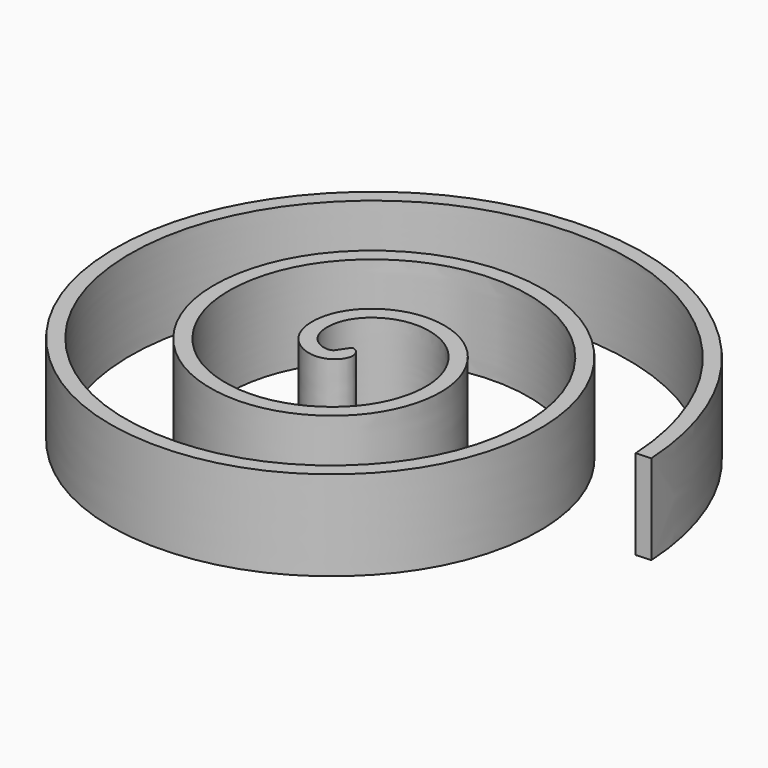
from build123d import *

# Parameters (mm, degrees)
F1_DEPTH = 3


# Not quite as in the source:
# - the dataset's text gives a spline's control points without its knots; the knots are read off the source's solid


with BuildPart() as f1:
    # F0 (on Top) → F1 (new body)
    with BuildSketch(Plane.XY):
        with BuildLine():
            Line((9.780739, 0.387732), (10.280037, 0.414221))
            add(Edge.make_bspline(
                [(10.280037, 0.414221), (10.201374, 1.896982), (9.787847, 3.342673), (7.912828, 6.782154), (5.908292, 8.419424), (1.404738, 9.873726), (-1.068266, 9.68826), (-5.152995, 7.729246), (-6.745094, 5.971338), (-8.285187, 1.926739), (-8.230102, -0.336088), (-6.637868, -4.142075), (-5.114518, -5.666794), (-1.522909, -7.245819), (0.523612, -7.296699), (4.02363, -6.032875), (5.460011, -4.730316), (7.03213, -1.581924), (7.164322, 0.244253), (6.1887, 3.414553), (5.091573, 4.743007), (2.372921, 6.26368), (0.769032, 6.452455), (-2.051397, 5.723262), (-3.253819, 4.81473), (-4.680076, 2.508754), (-4.900784, 1.127007), (-4.374962, -1.327091), (-3.636828, -2.386958), (-1.723014, -3.67766), (-0.561192, -3.905889), (1.513882, -3.53938), (2.41635, -2.952214), (3.53244, -1.406757), (3.74417, -0.4606), (3.492204, 1.226583), (3.035476, 1.958572), (1.831454, 2.863311), (1.094698, 3.035068), (-0.199589, 2.852457), (-0.749855, 2.504675), (-1.533897, 1.443211), (-1.550306, 0.6687), (-1.006795, -0.355611), (-0.483723, -0.590581), (0.31479, -0.499144), (0.565644, -0.199696), (0.587079, 0.257695), (0.437465, 0.414221), (0.280037, 0.414221)],
                knots=[0, 0, 0, 0, 0.444828, 0.444828, 1.20184, 1.20184, 1.958852, 1.958852, 2.715863, 2.715863, 3.472875, 3.472875, 4.229887, 4.229887, 4.986898, 4.986898, 5.74391, 5.74391, 6.500922, 6.500922, 7.257934, 7.257934, 8.014945, 8.014945, 8.771957, 8.771957, 9.528969, 9.528969, 10.28598, 10.28598, 11.042992, 11.042992, 11.800004, 11.800004, 12.557016, 12.557016, 13.314027, 13.314027, 14.071039, 14.071039, 14.828051, 14.828051, 15.871808, 15.871808, 16.915566, 16.915566, 17.959323, 17.959323, 18.849556, 18.849556, 18.849556, 18.849556], degree=3))
            Line((0.280037, 0.414221), (0, 0))
            add(Edge.make_bspline(
                [(9.780739, 0.387732), (9.74352, 1.0893), (9.627239, 1.782739), (9.190874, 3.327075), (8.818938, 4.159977), (7.408688, 6.3655), (6.072256, 7.52967), (3.743664, 8.6388), (2.873872, 8.894155), (1.109344, 9.129268), (0.215254, 9.111441), (-1.684864, 8.790436), (-2.674888, 8.429099), (-4.432872, 7.377766), (-5.205213, 6.692866), (-6.441686, 5.130602), (-6.908878, 4.257358), (-7.48617, 2.423193), (-7.601706, 1.462288), (-7.502539, -0.402135), (-7.294131, -1.305405), (-6.579773, -2.954878), (-6.075092, -3.703724), (-4.867311, -4.967602), (-4.167396, -5.48549), (-2.086789, -6.519112), (-0.582008, -6.730691), (1.497375, -6.415822), (2.148107, -6.213988), (3.347927, -5.630846), (3.898464, -5.251889), (4.974498, -4.259547), (5.462609, -3.612517), (6.155922, -2.210614), (6.363706, -1.45405), (6.505383, 0.061953), (6.439853, 0.820895), (5.909609, 2.733022), (5.188308, 3.794346), (3.764358, 4.944668), (3.205967, 5.252921), (2.03206, 5.662022), (1.417697, 5.764927), (0.236049, 5.769638), (-0.330291, 5.67946), (-1.385564, 5.325123), (-1.876581, 5.063109), (-2.832326, 4.344697), (-3.269252, 3.860145), (-3.904942, 2.787398), (-4.107783, 2.197187), (-4.284969, 0.990423), (-4.252084, 0.376095), (-3.952326, -0.757662), (-3.687948, -1.281657), (-3.051712, -2.105405), (-2.703086, -2.425822), (-1.93731, -2.91495), (-1.518825, -3.086644), (-0.582892, -3.30224), (-0.063637, -3.314353), (0.899903, -3.13575), (1.349435, -2.94605), (2.06902, -2.461715), (2.354125, -2.186037), (2.793433, -1.574326), (2.95069, -1.236114), (3.158615, -0.476271), (3.181727, -0.053218), (3.057244, 0.725661), (2.910747, 1.087483), (2.538565, 1.650708), (2.331618, 1.867296), (1.875955, 2.198462), (1.625236, 2.316159), (1.101938, 2.461474), (0.829253, 2.483139), (0.19368, 2.415006), (-0.153423, 2.256147), (-0.576967, 1.902955), (-0.702944, 1.746289), (-0.877599, 1.418506), (-0.928754, 1.245469), (-0.969026, 0.896639), (-0.95291, 0.721875), (-0.875692, 0.454849), (-0.824332, 0.355756), (-0.698624, 0.188184), (-0.624987, 0.121088), (-0.456411, 0.010296), (-0.359708, -0.026468), (-0.19386, -0.05676), (-0.131603, -0.050861), (-0.04901, -0.026879), (-0.02243, -0.014295), (0, 0)],
                knots=[0, 0, 0, 0, 0.221747, 0.221747, 0.512221, 0.512221, 1.073527, 1.073527, 1.377907, 1.377907, 1.682287, 1.682287, 2.047695, 2.047695, 2.413104, 2.413104, 2.772618, 2.772618, 3.132133, 3.132133, 3.484816, 3.484816, 3.837499, 3.837499, 4.185068, 4.185068, 4.795145, 4.795145, 5.089427, 5.089427, 5.383709, 5.383709, 5.747579, 5.747579, 6.111449, 6.111449, 6.474268, 6.474268, 7.093295, 7.093295, 7.428086, 7.428086, 7.762877, 7.762877, 8.08315, 8.08315, 8.403422, 8.403422, 8.790053, 8.790053, 9.176684, 9.176684, 9.574293, 9.574293, 9.971901, 9.971901, 10.309708, 10.309708, 10.647516, 10.647516, 11.051009, 11.051009, 11.454502, 11.454502, 11.802498, 11.802498, 12.150494, 12.150494, 12.566646, 12.566646, 12.982798, 12.982798, 13.328936, 13.328936, 13.675074, 13.675074, 14.040579, 14.040579, 14.604791, 14.604791, 14.960438, 14.960438, 15.316085, 15.316085, 15.695682, 15.695682, 16.006658, 16.006658, 16.317635, 16.317635, 16.682214, 16.682214, 17.046793, 17.046793, 17.271646, 17.271646, 17.271646, 17.271646], degree=3))
        make_face()
    extrude(amount=F1_DEPTH)


solid = f1.part
